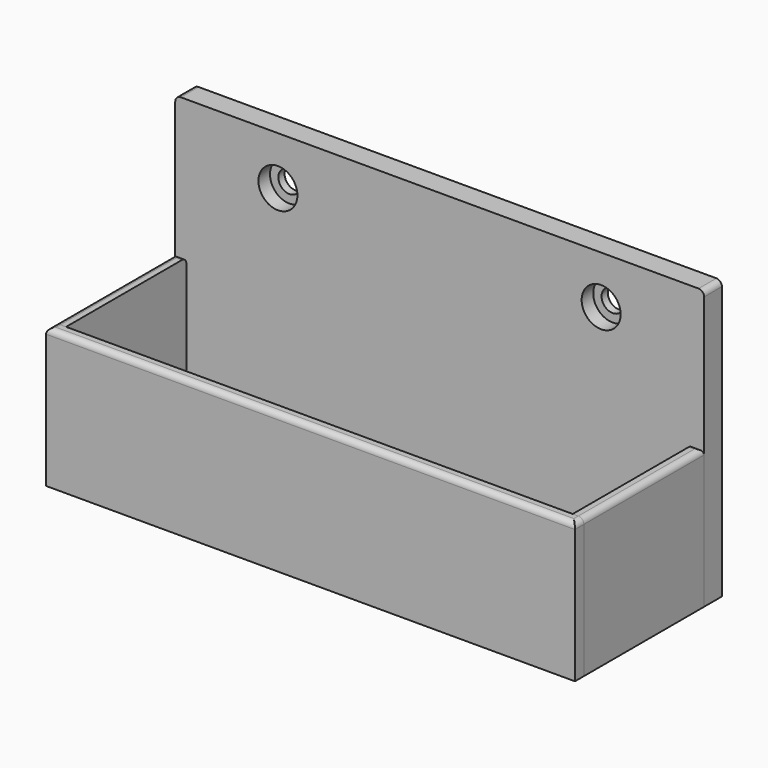
from build123d import *

# Parameters (mm, degrees)
F0_W      = 95
F0_H      = 33
F1_DEPTH  = 2
F4_W      = 95
F4_H      = 2
F7_DEPTH  = 25
F5_W      = 2
F5_H      = 27
F6_W      = 2
F6_H      = 27
F3_W      = 95
F3_H      = 4
F8_DEPTH  = 50
F2_W      = 52
F2_H      = 25
F9_DEPTH  = 6
F10_R     = 1
F10_2_R   = 1
F10_3_R   = 1
F10_4_R   = 1
F10_5_R   = 1
F11_R     = 2
F12_DEPTH = 4
F13_R     = 3.5
F14_DEPTH = 2.6


with BuildPart() as f1:
    # F0 (on Top) → F1 (new body)
    with BuildSketch(Plane.XY):
        Rectangle(F0_W, F0_H)
    extrude(amount=F1_DEPTH)

    # F2 (on face) → F9 (cut)
    with BuildSketch(Plane.XY):
        with Locations((0.9772641808, 0.0461841002)):
            Rectangle(F2_W, F2_H)
    extrude(amount=F9_DEPTH, mode=Mode.SUBTRACT)

    # F10
    f10_edges = [f1.edges().sort_by_distance(p)[0] for p in [
        (-47.5, 0, 0),
        (47.5, 0, 0),
        (0, -16.5, 0),
        (-25.022736, -12.453816, 1),
        (26.977264, -12.453816, 1),
        (26.977264, 12.546184, 1),
        (-25.022736, 12.546184, 1),
    ]]
    fillet(f10_edges, radius=F10_R)


with BuildPart() as f7:
    # F4 (on face) → F7 (new body)
    with BuildSketch(Plane.XY):
        with Locations((0, -15.5)):
            Rectangle(F4_W, F4_H)
    extrude(amount=F7_DEPTH)

    # F10#2
    f10_2_edges = [f7.edges().sort_by_distance(p)[0] for p in [
        (0, -16.5, 25),
        (-47.5, -15.5, 25),
        (47.5, -15.5, 25),
    ]]
    fillet(f10_2_edges, radius=F10_2_R)


with BuildPart() as f7b:
    # F5 (on face) → F7, piece 2 (new body)
    with BuildSketch(Plane.XY):
        with Locations((-46.5, -1)):
            Rectangle(F5_W, F5_H)
    extrude(amount=F7_DEPTH)

    # F10#3
    f10_3_edges = [f7b.edges().sort_by_distance(p)[0] for p in [
        (-46.5, 12.5, 25),
        (-47.5, -1, 25),
    ]]
    fillet(f10_3_edges, radius=F10_3_R)


with BuildPart() as f7c:
    # F6 (on face) → F7, piece 3 (new body)
    with BuildSketch(Plane.XY):
        with Locations((46.5, -1)):
            Rectangle(F6_W, F6_H)
    extrude(amount=F7_DEPTH)

    # F10#4
    f10_4_edges = [f7c.edges().sort_by_distance(p)[0] for p in [
        (46.5, 12.5, 25),
        (47.5, -1, 25),
    ]]
    fillet(f10_4_edges, radius=F10_4_R)


with BuildPart() as f8:
    # F3 (on face) → F8 (new body)
    with BuildSketch(Plane.XY):
        with Locations((0, 14.5)):
            Rectangle(F3_W, F3_H)
    extrude(amount=F8_DEPTH)

    # F10#5
    f10_5_edges = [f8.edges().sort_by_distance(p)[0] for p in [
        (47.5, 14.5, 50),
        (-47.5, 14.5, 50),
        (-47.5, 14.5, 0),
    ]]
    fillet(f10_5_edges, radius=F10_5_R)

    # F11 (on face) → F12 (cut)
    with BuildSketch(Plane.XZ.offset(-12.5)):
        with Locations((-29.0568154305, 41.3045398891)):
            Circle(F11_R)
        with Locations((29.0029011667, 41.3656570017)):
            Circle(F11_R)
    extrude(amount=-F12_DEPTH, mode=Mode.SUBTRACT)

    # F13 (on face) → F14 (cut)
    with BuildSketch(Plane.XZ.offset(-12.5)):
        with Locations((-29.0568154305, 41.3045398891)):
            Circle(F13_R)
        with Locations((29.0029011667, 41.3656570017)):
            Circle(F13_R)
    extrude(amount=-F14_DEPTH, mode=Mode.SUBTRACT)


solid = Compound([f1.part, f7.part, f7b.part, f7c.part, f8.part])
